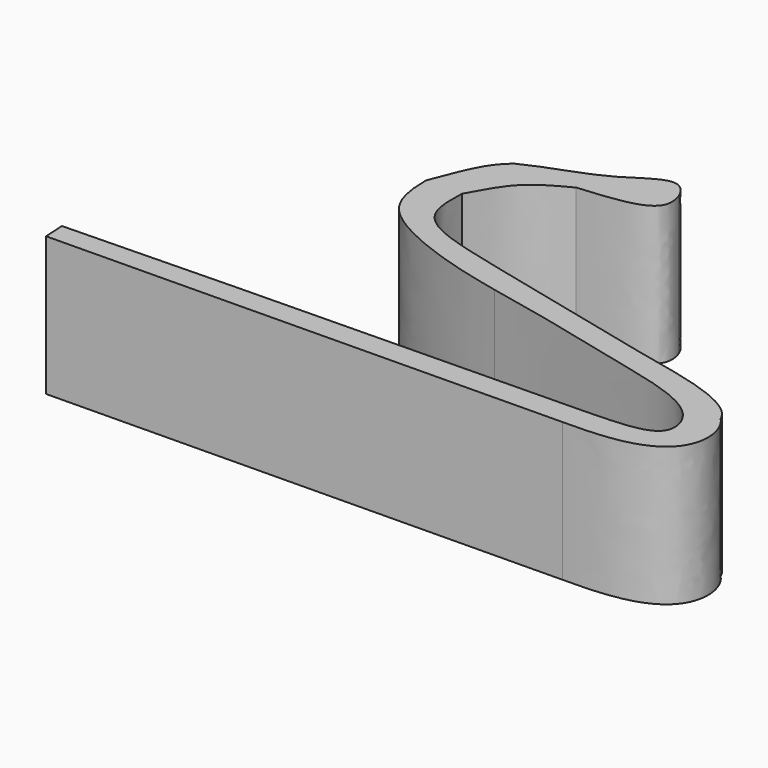
from build123d import *

# Parameters (mm, degrees)
F1_DEPTH = 25


with BuildPart() as f1:
    # F0 (on Top) → F1 (new body)
    with BuildSketch(Plane.XY):
        with BuildLine():
            add(Edge.make_bspline(
                [(-21.8713730574, 11.7478426546), (-24.6937042664, 9.4094434093), (-25.8700233112, 6.5320717403), (-28.3579751849, 0)],
                knots=[0.8208595676, 0.8208595676, 0.8208595676, 0.8208595676, 1, 1, 1, 1], degree=3))
            add(Edge.make_bspline(
                [(-28.3579751849, 0), (-28.3579751849, -6.1687799171), (-25.0409646378, -12.0046337294), (-10.0117255998, -17.7891546067), (-3.2871411917, -19.2140408192), (0, -19.9794825166)],
                knots=[0, 0, 0, 0, 0.331420671, 0.694447253, 1, 1, 1, 1], degree=3))
            add(Edge.make_bspline(
                [(0, -19.9794825166), (3.2359946593, -20.639355481), (10.6923897216, -22.1620353004), (27.3092514073, -26.421313522), (44.5848104203, -30.2222938762), (47.4136166373, -40.5343330295), (30.574815433, -41.1091785279), (-10.8965561329, -41.6940459683), (-28.7263703833, -42.0510822643), (-48.5938647815, -42.5227759959), (-59.6622340381, -42.8131781518)],
                knots=[0, 0, 0, 0, 0.0950500628, 0.2192239412, 0.3403780873, 0.4127924201, 0.5196375059, 0.7105447801, 0.8386423011, 1, 1, 1, 1], degree=3))
            Line((-59.6622340381, -42.8131781518), (-59.4390779734, -46.6422252357))
            Line((-59.4390779734, -46.6422252357), (32.6148234308, -45.4555265605))
            add(Edge.make_bspline(
                [(49.2732562125, -30.7161379606), (51.6651031243, -33.289034819), (52.2331081198, -39.9179667879), (45.1377357024, -45.147660188), (36.7909185588, -45.4555265605), (32.6148234308, -45.4555265605)],
                knots=[0, 0, 0, 0, 0.3185407776, 0.6171943595, 1, 1, 1, 1], degree=3))
            add(Edge.make_bspline(
                [(-21.8713730574, 0), (-21.9722817567, -2.8763830867), (-22.1773484336, -9.4915970364), (-8.0406845901, -13.6383181356), (10.633621372, -17.7842417202), (27.4880945573, -22.2413088232), (47.3097975389, -26.0467778065), (49.2732562125, -30.7161379606)],
                knots=[0, 0, 0, 0, 0.1422401643, 0.3222214996, 0.5428511495, 0.7661439075, 1, 1, 1, 1], degree=3))
            add(Edge.make_bspline(
                [(-21.8713730574, 0), (-19.7871929363, 3.8302198486), (-17.7091250818, 7.2460366741), (-14.0928466211, 9.6460624163), (-10.5021484196, 11.5007823333)],
                knots=[0, 0, 0, 0, 0.1414458784, 0.2810663656, 0.2810663656, 0.2810663656, 0.2810663656], degree=3))
            add(Edge.make_bspline(
                [(-10.5021484196, 11.5007823333), (-6.1301731241, 13.7590589141), (0.9018725283, 16.9994990971), (2.360772568, 18.4400047566)],
                knots=[0.2810663656, 0.2810663656, 0.2810663656, 0.2810663656, 0.4510659832, 0.4510659832, 0.4510659832, 0.4510659832], degree=3))
            add(Edge.make_bspline(
                [(2.0079142252, 19.2091199353), (2.1421984622, 18.9628385703), (2.2606148291, 18.7045079104), (2.360772568, 18.4400047566)],
                knots=[0.6103989723, 0.6103989723, 0.6103989723, 0.6103989723, 0.6334231998, 0.6334231998, 0.6334231998, 0.6334231998], degree=3))
            add(Edge.make_bspline(
                [(2.0079142252, 19.2091199353), (0.3720880298, 19.397415037), (-4.1983607486, 18.5614293228), (-8.2476707175, 17.5434458946)],
                knots=[0.5030943267, 0.5030943267, 0.5030943267, 0.5030943267, 0.6326984682, 0.6326984682, 0.6326984682, 0.6326984682], degree=3))
            add(Edge.make_bspline(
                [(-21.8713730574, 11.7478426546), (-16.8125833414, 14.249205109), (-12.3075685491, 15.2426061849), (-8.2476707175, 17.5434458946)],
                knots=[0, 0, 0, 0, 0.2953761193, 0.2953761193, 0.2953761193, 0.2953761193], degree=3))
        make_face()
        with BuildLine():
            add(Edge.make_bspline(
                [(-8.2476707175, 17.5434458946), (-5.0822698034, 19.3373531362), (-1.1224608688, 22.8784119697), (1.5137697263, 20.1153959386), (2.0079142252, 19.2091199353)],
                knots=[0.2953761193, 0.2953761193, 0.2953761193, 0.2953761193, 0.5256735003, 0.6103989723, 0.6103989723, 0.6103989723, 0.6103989723], degree=3))
            add(Edge.make_bspline(
                [(2.0079142252, 19.2091199353), (0.3720880298, 19.397415037), (-4.1983607486, 18.5614293228), (-8.2476707175, 17.5434458946)],
                knots=[0.5030943267, 0.5030943267, 0.5030943267, 0.5030943267, 0.6326984682, 0.6326984682, 0.6326984682, 0.6326984682], degree=3))
        make_face()
        with BuildLine():
            add(Edge.make_bspline(
                [(2.360772568, 18.4400047566), (2.7160561786, 17.5017483973), (3.2795126261, 12.9418978403), (-2.9351401887, 12.1017342069), (-10.5021484196, 11.5007823333)],
                knots=[0.6334231998, 0.6334231998, 0.6334231998, 0.6334231998, 0.7150956774, 1, 1, 1, 1], degree=3))
            add(Edge.make_bspline(
                [(-10.5021484196, 11.5007823333), (-6.1301731241, 13.7590589141), (0.9018725283, 16.9994990971), (2.360772568, 18.4400047566)],
                knots=[0.2810663656, 0.2810663656, 0.2810663656, 0.2810663656, 0.4510659832, 0.4510659832, 0.4510659832, 0.4510659832], degree=3))
        make_face()
    extrude(amount=F1_DEPTH)


solid = f1.part
